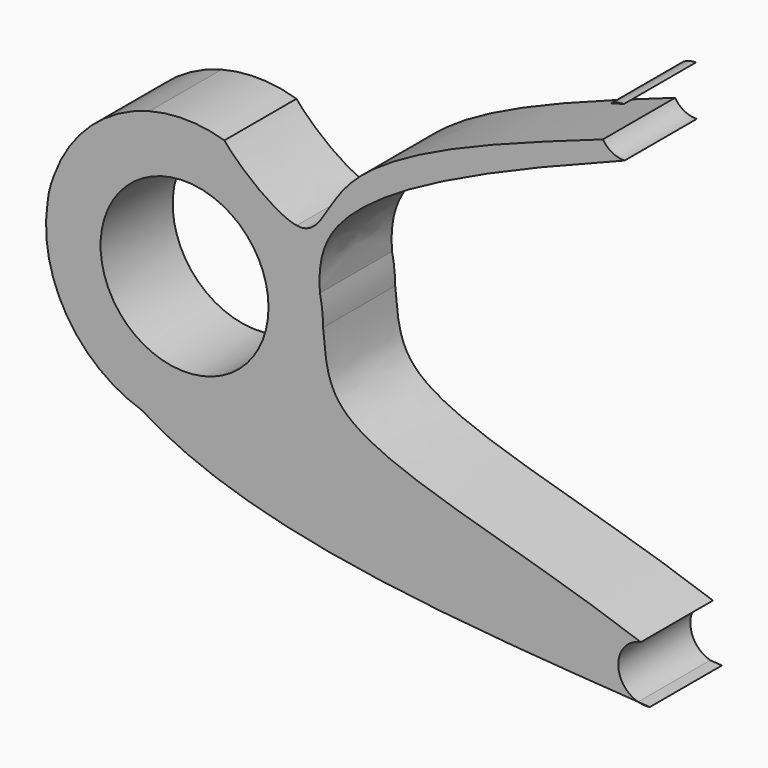
from build123d import *

# Parameters (mm, degrees)
F1_DEPTH = 25.4
F0_R     = 23.6593869312


with BuildPart() as f1:
    # F0 (on Front) → F1 (new body)
    with BuildSketch(Plane.XZ):
        with BuildLine():
            add(Edge.make_bspline(
                [(75.9254321456, 83.0235277666), (74.7294280544, 82.6927874869), (73.5334280539, 82.3620352717), (72.3376928193, 82.0312405203)],
                knots=[0, 0, 0, 0, 0.0073316061, 0.0073316061, 0.0073316061, 0.0073316061], degree=3))
            ThreePointArc((75.9254321456, 83.0235277666), (74.0642156447, 82.7708851046), (72.3376928194, 82.0312405203))
        make_face()
    extrude(amount=F1_DEPTH)


with BuildPart() as f1b:
    # F0 (on Front) → F1, piece 2 (new body)
    with BuildSketch(Plane.XZ):
        with BuildLine():
            add(Edge.make_bspline(
                [(76.1346470657, 69.0624530107), (40.7292389403, 55.4358728105), (-8.4882690711, 35.1479862328), (-10.0969930291, 13.5229108802), (-9.7391861118, 8.2574256301)],
                knots=[0, 0, 0, 0, 0.3400525355, 0.4531553438, 0.4531553438, 0.4531553438, 0.4531553438], degree=3))
            ThreePointArc((76.1346470657, 69.0624530107), (72.6443374796, 69.8782898329), (70.0187498647, 72.3184005689))
            add(Edge.make_bspline(
                [(-16.28206518, 22.9048247821), (-15.9978816605, 22.8614061319), (-9.847888416, 22.2541104927), (-4.9630436623, 45.7648826483), (39.9145521125, 61.6532519518), (70.0187498647, 72.3184005689)],
                knots=[0.6107795309, 0.6107795309, 0.6107795309, 0.6107795309, 0.6167186955, 0.7430558298, 1, 1, 1, 1], degree=3))
            ThreePointArc((-16.28206518, 22.9048247821), (-12.2500691202, 15.9208598799), (-9.7391861118, 8.2574256301))
        make_face()
        with BuildLine():
            add(Edge.make_bspline(
                [(-9.7391861118, 8.2574256301), (-9.5488772889, 5.4568417072), (-9.1437609317, 2.6935729525), (-8.8558278998, 0)],
                knots=[0.4531553438, 0.4531553438, 0.4531553438, 0.4531553438, 0.513311985, 0.513311985, 0.513311985, 0.513311985], degree=3))
            ThreePointArc((-9.7391861118, 8.2574256301), (-12.2500691202, 15.9208598799), (-16.28206518, 22.9048247821))
            add(Edge.make_bspline(
                [(-36.6569671608, 37.3842575617), (-34.0559655004, 33.839361088), (-22.9517472418, 23.9238444403), (-16.28206518, 22.9048247821)],
                knots=[0.4713895345, 0.4713895345, 0.4713895345, 0.4713895345, 0.6107795309, 0.6107795309, 0.6107795309, 0.6107795309], degree=3))
            ThreePointArc((-36.6569671608, 37.3842575617), (-47.1995868952, 39.0297823491), (-57.7939230416, 37.7591036685))
            add(Edge.make_bspline(
                [(-57.7939230416, 37.7591036685), (-71.2879137352, 30.3920746047), (-80.7433533788, 22.546843239), (-84.6419629659, 13.1614831137)],
                knots=[0.3158866582, 0.3158866582, 0.3158866582, 0.3158866582, 0.4548873169, 0.4548873169, 0.4548873169, 0.4548873169], degree=3))
            ThreePointArc((-84.6419629659, 13.1614831137), (-85.7657136885, 9.453341157), (-86.5163145506, 5.6520610039))
            add(Edge.make_bspline(
                [(-86.5163145506, 5.6520610039), (-87.8220049343, -8.256393814), (-78.1636088875, -25.5056272441), (-59.8753358981, -37.1509972704)],
                knots=[0.4903848461, 0.4903848461, 0.4903848461, 0.4903848461, 0.6791592516, 0.6791592516, 0.6791592516, 0.6791592516], degree=3))
            ThreePointArc((-59.8753358981, -37.1509972704), (-24.9133595896, -31.5562465868), (-8.8558278998, 0))
        make_face()
        with Locations((-47.8917472064, 0)):
            Circle(F0_R, mode=Mode.SUBTRACT)
        with BuildLine():
            ThreePointArc((-8.8558278998, 0), (-9.0772956945, 4.1522704562), (-9.7391861118, 8.2574256301))
            add(Edge.make_bspline(
                [(-9.7391861118, 8.2574256301), (-9.5488772889, 5.4568417072), (-9.1437609317, 2.6935729525), (-8.8558278998, 0)],
                knots=[0.4531553438, 0.4531553438, 0.4531553438, 0.4531553438, 0.513311985, 0.513311985, 0.513311985, 0.513311985], degree=3))
        make_face()
        with BuildLine():
            add(Edge.make_bspline(
                [(-57.7939230416, 37.7591036685), (-71.2879137352, 30.3920746047), (-80.7433533788, 22.546843239), (-84.6419629659, 13.1614831137)],
                knots=[0.3158866582, 0.3158866582, 0.3158866582, 0.3158866582, 0.4548873169, 0.4548873169, 0.4548873169, 0.4548873169], degree=3))
            ThreePointArc((-57.7939230416, 37.7591036685), (-74.2616570397, 28.7824747286), (-84.6419629659, 13.1614831137))
        make_face()
        with BuildLine():
            add(Edge.make_bspline(
                [(-8.8558278998, 0), (-8.1092874361, -6.9837808721), (-8.2378825667, -27.3137566504), (44.0538892813, -35.7910694427), (80.699708097, -48.9266225955)],
                knots=[0.513311985, 0.513311985, 0.513311985, 0.513311985, 0.669283554, 1, 1, 1, 1], degree=3))
            ThreePointArc((-8.8558278998, 0), (-24.9133595896, -31.5562465868), (-59.8753358981, -37.1509972704))
            add(Edge.make_bspline(
                [(-59.8753358981, -37.1509972704), (-29.4016014528, -56.5556678974), (25.033443589, -60.4009148555), (79.9312097407, -64.0020462349)],
                knots=[0.6791592516, 0.6791592516, 0.6791592516, 0.6791592516, 0.9937138904, 0.9937138904, 0.9937138904, 0.9937138904], degree=3))
            ThreePointArc((79.9312097407, -64.0020462349), (74.3325035366, -56.1593418997), (80.699708097, -48.9266225955))
        make_face()
        with BuildLine():
            ThreePointArc((-86.5163145506, 5.6520610039), (-85.7657136885, 9.453341157), (-84.6419629659, 13.1614831137))
            add(Edge.make_bspline(
                [(-84.6419629659, 13.1614831137), (-85.637577009, 10.7646808353), (-86.2707898333, 8.2674355824), (-86.5163145506, 5.6520610039)],
                knots=[0.4548873169, 0.4548873169, 0.4548873169, 0.4548873169, 0.4903848461, 0.4903848461, 0.4903848461, 0.4903848461], degree=3))
        make_face()
        with BuildLine():
            ThreePointArc((-86.5163145506, 5.6520610039), (-81.0326858435, -20.6271952134), (-59.8753358981, -37.1509972704))
            add(Edge.make_bspline(
                [(-86.5163145506, 5.6520610039), (-87.8220049343, -8.256393814), (-78.1636088875, -25.5056272441), (-59.8753358981, -37.1509972704)],
                knots=[0.4903848461, 0.4903848461, 0.4903848461, 0.4903848461, 0.6791592516, 0.6791592516, 0.6791592516, 0.6791592516], degree=3))
        make_face()
    extrude(amount=F1_DEPTH)


with BuildPart() as f1c:
    # F0 (on Front) → F1, piece 3 (new body)
    with BuildSketch(Plane.XZ):
        with BuildLine():
            add(Edge.make_bspline(
                [(79.9312097407, -64.0020462349), (81.0282953659, -64.0740118129), (82.1255657864, -64.1458798992), (83.2228334599, -64.2177727256)],
                knots=[0.9937138904, 0.9937138904, 0.9937138904, 0.9937138904, 1, 1, 1, 1], degree=3))
            ThreePointArc((79.9312097407, -64.0020462349), (81.5654106231, -64.2870734798), (83.2228334599, -64.2177727256))
        make_face()
    extrude(amount=F1_DEPTH)


solid = Compound([f1.part, f1b.part, f1c.part])
